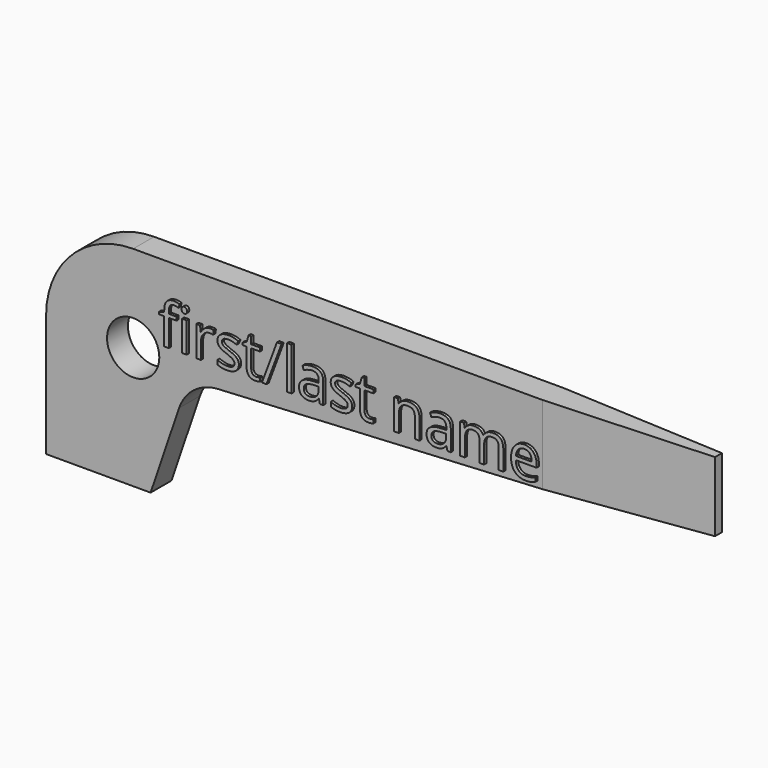
from build123d import *

# Parameters (mm, degrees)
F1_DEPTH     = 2.38125
F2_R         = 2.38125
F3_DEPTH     = 25.4
F5_DEPTH     = 25.4
F6_TEXT_SIZE = 5.1457680658
F7_DEPTH     = 0.254


# Not quite as in the source:
# - Text() gives the source's letters only with a copy of the font that has no kerning and outlines rounded to 1/6400 em; it was checked with that copy


with BuildPart() as f1:
    # F0 (on Front) → F1 (new body)
    with BuildSketch(Plane.XZ):
        with BuildLine():
            Line((60.325, 19.05), (7.9375, 19.05))
            ThreePointArc((7.9375, 19.05), (2.3248399243, 16.7251600757), (0, 11.1125))
            Line((0, 11.1125), (0, 0))
            Line((0, 0), (9.525, 0))
            Line((9.525, 0), (12.1173647876, 7.6271664624))
            ThreePointArc((12.1173647876, 7.6271664624), (13.4786145605, 9.5135918491), (15.6631963617, 10.3130942181))
            Line((15.6631963617, 10.3130942181), (60.325, 12.7))
            Line((60.325, 12.7), (60.325, 19.05))
        make_face()
    extrude(amount=F1_DEPTH)

    # F2 (on face) → F3 (cut)
    with BuildSketch(Plane.XZ.offset(2.38125)):
        with Locations((7.9375, 11.1125)):
            Circle(F2_R)
    extrude(amount=-F3_DEPTH, mode=Mode.SUBTRACT)

    # F4 (on face) → F5 (cut)
    with BuildSketch(Plane.XY.offset(19.05)):
        Polygon((60.325, -2.38125), (60.325, -1.5875), (45.24375, -2.38125), align=None)
        Polygon((60.325, 0), (45.24375, 0), (60.325, -0.79375), align=None)
    extrude(amount=-F5_DEPTH, mode=Mode.SUBTRACT)

    # F6 (on face) → F7 (join)
    with BuildSketch(Plane.XZ.offset(2.38125)):
        with Locations((10.4077042206, 12.3035097495)):
            Text('first/last name', F6_TEXT_SIZE, font='Open Sans', text_align=(TextAlign.LEFT, TextAlign.BOTTOM))
    extrude(amount=F7_DEPTH)


solid = f1.part
